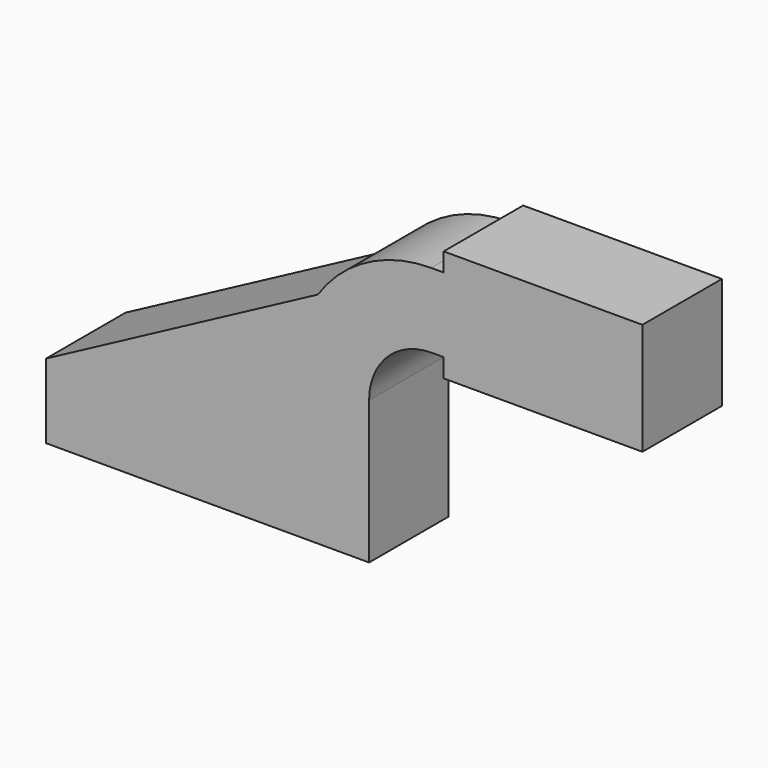
from build123d import *

# Parameters (mm, degrees)
F1_DEPTH = 25.4


# Not quite as in the source:
# - a feature names something its author has since deleted; it is built from what else it names


with BuildPart() as f1:
    # F0 (on Front) → F1 (new body)
    with BuildSketch(Plane.XZ):
        Polygon((-41.275, -9.525), (41.275, -9.525), (41.275, 9.525), (22.225, 9.525), (-41.275, 9.525), align=None)
        with BuildLine():
            Line((22.225, 9.525), (41.275, 9.525))
            Line((41.275, 9.525), (41.275, 27.0002))
            ThreePointArc((41.275, 27.0002), (45.9246798487, 38.2255201513), (57.15, 42.8752))
            Line((57.15, 42.8752), (60.325, 42.8752))
            Line((60.325, 42.8752), (60.325, 61.9252))
            Line((60.325, 61.9252), (57.15, 61.9252))
            add(Edge.make_bspline(
                [(57.15, 61.9252), (47.4917497752, 56.7832722029), (37.8334995503, 51.6413444058), (28.1752493255, 46.4994166087)],
                knots=[0, 0, 0, 0, 32.8251575759, 32.8251575759, 32.8251575759, 32.8251575759], degree=3))
            ThreePointArc((28.1752493255, 46.4994166087), (23.7456680032, 37.1936404813), (22.225, 27.0002))
            Line((22.225, 27.0002), (22.225, 9.525))
        make_face()
        with BuildLine():
            add(Edge.make_bspline(
                [(28.1752493255, 46.4994166087), (5.025166217, 34.1746110724), (-18.1249168915, 21.8498055362), (-41.275, 9.525)],
                knots=[32.8251575759, 32.8251575759, 32.8251575759, 32.8251575759, 111.5045361635, 111.5045361635, 111.5045361635, 111.5045361635], degree=3))
            Line((-41.275, 9.525), (22.225, 9.525))
            Line((22.225, 9.525), (22.225, 27.0002))
            ThreePointArc((22.225, 27.0002), (23.7456680032, 37.1936404813), (28.1752493255, 46.4994166087))
        make_face()
        with BuildLine():
            ThreePointArc((57.15, 61.9252), (40.737421212, 57.8284805639), (28.1752493255, 46.4994166087))
            add(Edge.make_bspline(
                [(57.15, 61.9252), (47.4917497752, 56.7832722029), (37.8334995503, 51.6413444058), (28.1752493255, 46.4994166087)],
                knots=[0, 0, 0, 0, 32.8251575759, 32.8251575759, 32.8251575759, 32.8251575759], degree=3))
        make_face()
        Polygon((60.325, 61.9252), (60.325, 42.8752), (60.325, 38.1), (111.125, 38.1), (111.125, 66.675), (60.325, 66.675), align=None)
    extrude(amount=F1_DEPTH)


solid = f1.part
